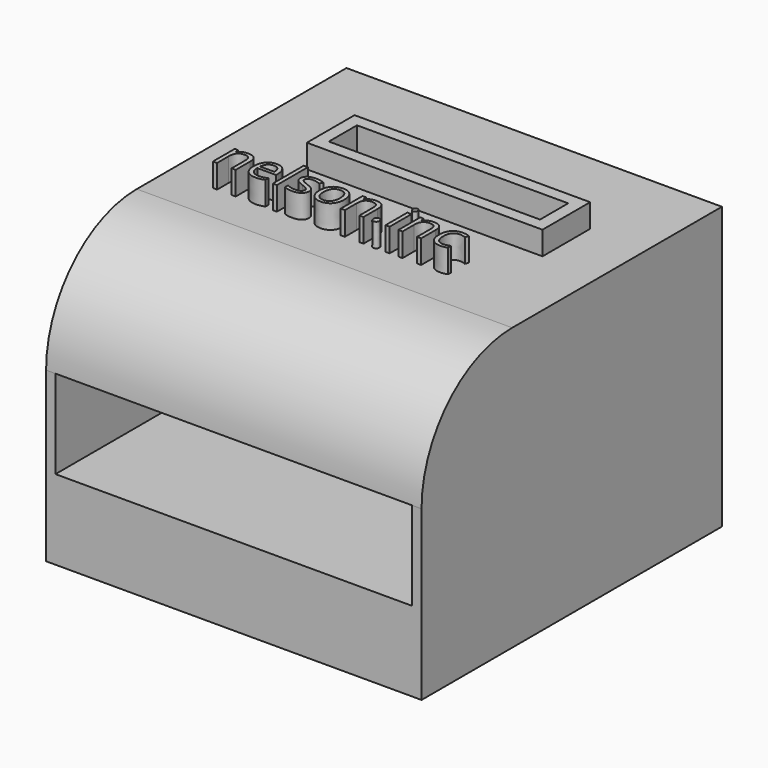
from build123d import *

# Parameters (mm, degrees)
F0_W         = 101.6
F0_H         = 101.6
F1_DEPTH     = 76.2
F2_R         = 30.6605122421
F3_T         = -2.54
F5_W         = 63.7540014073
F5_H         = 16.1290014073
F5_W_2       = 57.15
F5_H_2       = 9.525
F6_DEPTH     = 6.35
F7_TEXT_SIZE = 13.7800581752
F8_DEPTH     = 6.35
F9_W         = 52.0700009152
F9_H         = 4.4450009152
F10_DEPTH    = 2.794
F11_DEPTH    = 19.05


# Not quite as in the source:
# - a shell that OpenCascade refuses in one call is made with other operations: the cavity is built on its own and cut out
# - Text() gives the source's letters only with a copy of the font that has no kerning and outlines rounded to 1/6400 em; it was checked with that copy


with BuildPart() as f1:
    # F0 (on Top) → F1 (new body)
    with BuildSketch(Plane.XY):
        with Locations((-25.9461284995, -22.7656619072)):
            Rectangle(F0_W, F0_H)
    extrude(amount=F1_DEPTH)

    # F2
    f2_edges = [f1.edges().sort_by_distance(p)[0] for p in [
        (-25.946128, -73.565662, 76.2),
    ]]
    fillet(f2_edges, radius=F2_R)

    # F3: a shell. OpenCascade refuses it in one call, so the cavity is built on its own and cut out:
    # the body offset inwards by the wall thickness, plus a prism from it out through each open face.
    f3_core = offset(f1.part, amount=F3_T, mode=Mode.PRIVATE)
    f3_exits = [f3_core.faces().sort_by_distance(p)[0] for p in [
        (-25.946128, -71.025662, 24.039744),
    ]]
    add(f3_core, mode=Mode.SUBTRACT)
    extrude(f3_exits, amount=-F3_T, mode=Mode.SUBTRACT)

    # F5 (on face) → F6 (join)
    with BuildSketch(Plane.XY.offset(76.2)):
        with Locations((-22.4418110408, -5.3239395499)):
            Rectangle(F5_W, F5_H)
        with Locations((-22.4418110408, -5.3239395499)):
            Rectangle(F5_W_2, F5_H_2, mode=Mode.SUBTRACT)
    extrude(amount=F6_DEPTH)

    # F7 (on face) → F8 (join)
    with BuildSketch(Plane.XY.offset(76.2)):
        with Locations((-65.6361395959, -32.4878057986)):
            Text('nelson.inc', F7_TEXT_SIZE, font='Open Sans', text_align=(TextAlign.LEFT, TextAlign.BOTTOM))
    extrude(amount=F8_DEPTH)

    # F9 (on face) → F10 (join)
    with BuildSketch(Plane.XY.offset(76.2)):
        with Locations((-22.4418110408, -5.3239395499)):
            Rectangle(F9_W, F9_H)
    extrude(amount=-F10_DEPTH)

    # F11 (add): a face of the model
    f11_faces = [f1.faces().sort_by_distance(p)[0] for p in [
        (-25.9461284995, -24.0356619072, 2.54),
    ]]
    extrude(f11_faces, amount=F11_DEPTH)


solid = f1.part
